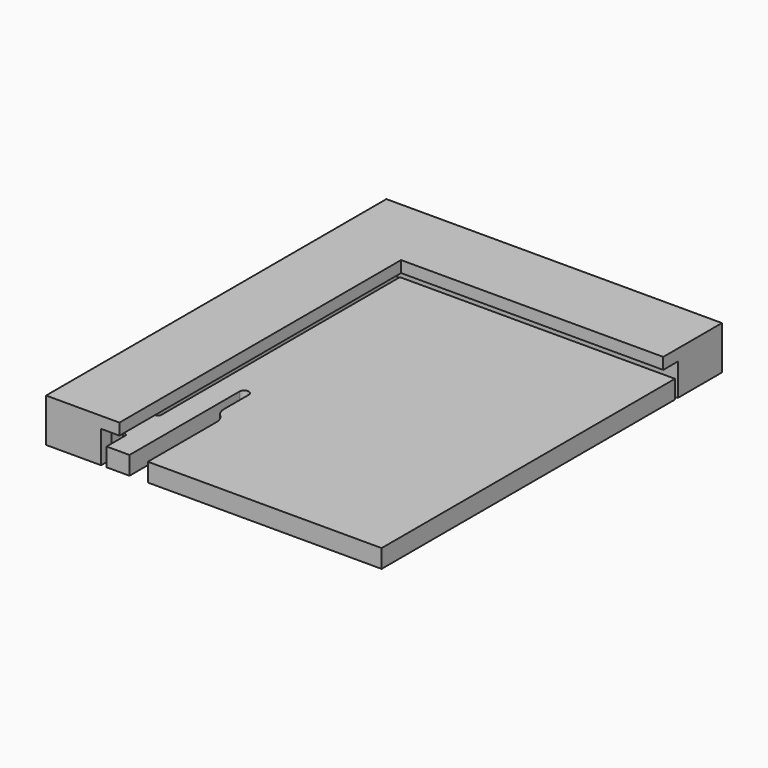
from build123d import *

# Parameters (mm, degrees)
F1_DEPTH = 1.27
F3_DEPTH = 2.2225
F5_DEPTH = 0.79375


# Not quite as in the source:
# - a feature of the source that left no trace in its solid (it failed there, or was rolled back) is left out


with BuildPart() as f1:
    # F0 (on Top) → F1 (new body)
    with BuildSketch(Plane.XY):
        with BuildLine():
            Line((0, -25.4), (0, 0))
            Line((0, 0), (-19.05, 0))
            Line((-19.05, 0), (-19.05, -20.7700322169))
            ThreePointArc((-19.05, -20.7700322169), (-20.0025, -22.225), (-19.05, -23.6799677831))
            Line((-19.05, -23.6799677831), (-19.05, -25.4))
            Line((-19.05, -25.4), (-17.4625, -25.4))
            Line((-17.4625, -25.4), (-17.4625, -15.875))
            ThreePointArc((-17.4625, -15.875), (-17.145, -15.5575), (-16.8275, -15.875))
            Line((-16.8275, -15.875), (-16.8275, -18.0204615818))
            ThreePointArc((-16.8275, -18.0204615818), (-16.7549952547, -18.3849675512), (-16.5485192091, -18.6939807909))
            Line((-16.5485192091, -18.6939807909), (-16.4714807909, -18.7710192091))
            ThreePointArc((-16.4714807909, -18.7710192091), (-16.2650047453, -19.0800324488), (-16.1925, -19.4445384182))
            Line((-16.1925, -19.4445384182), (-16.1925, -25.4))
            Line((-16.1925, -25.4), (0, -25.4))
        make_face()
    extrude(amount=F1_DEPTH)


with BuildPart() as f3:
    # F2 (on Top) → F3 (new body)
    with BuildSketch(Plane.XY):
        Polygon((-23.241, -25.4), (-19.431, -25.4), (-19.431, -24.5054677831), (-20.0025, -23.9339677831), (-20.0025, -20.7700322169), (-19.431, -20.7700322169), (-19.431, 0.254), (0, 0.254), (0, 4.064), (-23.241, 4.064), align=None)
    extrude(amount=F3_DEPTH)

    # F4 (on face) → F5 (join)
    with BuildSketch(Plane.XY.offset(2.2225)):
        Polygon((0, -1.016), (0, 4.064), (-23.241, 4.064), (-23.241, -25.4), (-18.161, -25.4), (-18.161, -1.016), align=None)
    extrude(amount=F5_DEPTH)


solid = Compound([f1.part, f3.part])
